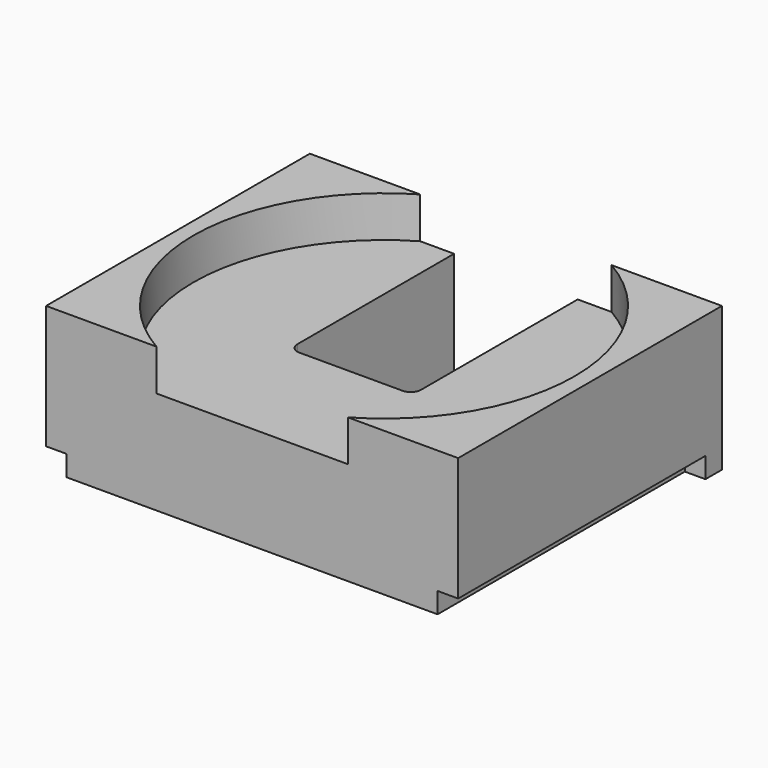
from build123d import *

# Parameters (mm, degrees)
F0_W          = 200
F0_H          = 160
F1_DEPTH      = 50
F3_DEPTH      = 20
F5_W          = 60
F5_H          = 120
F6_DEPTH      = 90
F6_DEPTH_BACK = 20
F9_W          = 10
F9_H          = 10
F10_DEPTH     = 150
F11_R         = 5


with BuildPart() as f1:
    # F0 (on Top) → F1 (new body)
    with BuildSketch(Plane.XY):
        Rectangle(F0_W, F0_H)
    extrude(amount=F1_DEPTH)

    # F2 (on face) → F3 (join)
    with BuildSketch(Plane.XY.offset(50)):
        with BuildLine():
            ThreePointArc((46.4354390525, 80), (80.1608636192, 46.1571873474), (92.5, 0))
            ThreePointArc((92.5, 0), (80.1608636192, -46.1571873474), (46.4354390525, -80))
            Line((46.4354390525, -80), (100, -80))
            Line((100, -80), (100, 80))
            Line((100, 80), (46.4354390525, 80))
        make_face()
        with BuildLine():
            ThreePointArc((-46.4354390525, -80), (-92.5, 0), (-46.4354390525, 80))
            Line((-46.4354390525, 80), (-100, 80))
            Line((-100, 80), (-100, -80))
            Line((-100, -80), (-46.4354390525, -80))
        make_face()
    extrude(amount=F3_DEPTH)

    # F5 (on Front) → F6 (cut, two sides)
    with BuildSketch(Plane.XZ) as f6_sk:
        Rectangle(F5_W, F5_H)
    extrude(amount=-F6_DEPTH, mode=Mode.SUBTRACT)
    extrude(f6_sk.sketch, amount=F6_DEPTH_BACK, mode=Mode.SUBTRACT)

    # F9 (on face) → F10 (cut)
    with BuildSketch(Plane.XZ.offset(80)):
        with Locations((95, 5)):
            Rectangle(F9_W, F9_H)
        with Locations((-95, 5)):
            Rectangle(F9_W, F9_H)
    extrude(amount=-F10_DEPTH, mode=Mode.SUBTRACT)

    # F11
    f11_edges = [f1.edges().sort_by_distance(p)[0] for p in [
        (-30, -20, 25),
        (30, -20, 25),
    ]]
    fillet(f11_edges, radius=F11_R)


solid = f1.part
